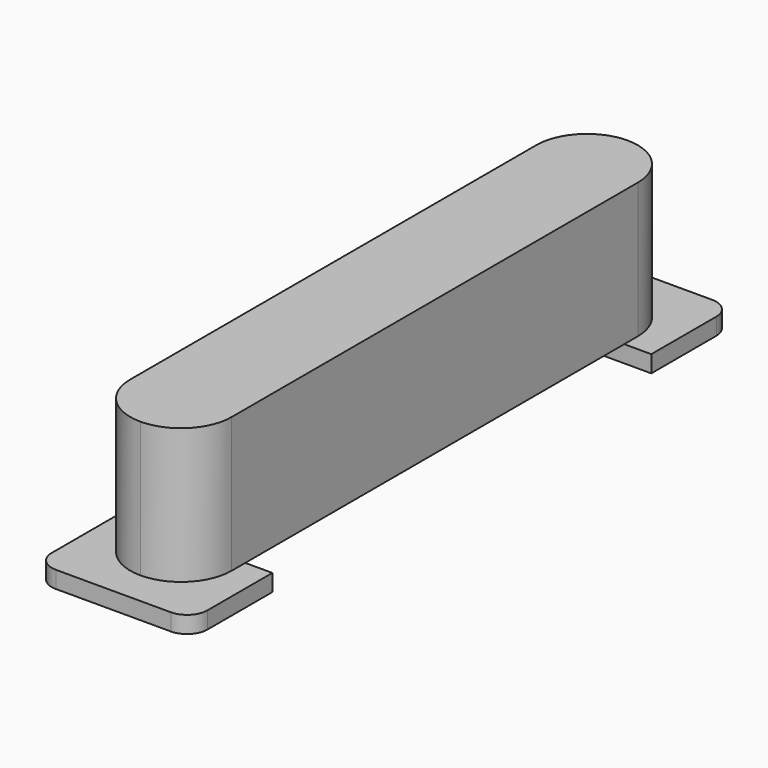
from build123d import *

# Parameters (mm, degrees)
F0_W     = 1.5
F0_H     = 1
F0_H_2   = 7
F1_DEPTH = 2
F2_DEPTH = 0.25
F3_R     = 0.74999
F4_R     = 0.3


# Not quite as in the source:
# - a fillet or chamfer is up to 0.001 mm smaller than in the source, because OpenCascade refuses the exact size
# - a feature names something its author has since deleted; it is built from what else it names


with BuildPart() as f1:
    # F0 (on Top) → F1 (new body)
    with BuildSketch(Plane.XY):
        with Locations((-0.75, 9.1787409857)):
            Rectangle(F0_W, F0_H)
        with Locations((-0.75, 5.1787409857)):
            Rectangle(F0_W, F0_H_2)
        with Locations((-0.75, 1.1787409857)):
            Rectangle(F0_W, F0_H)
    extrude(amount=F1_DEPTH)

    # F0 (on Top) → F2 (join)
    with BuildSketch(Plane.XY):
        with Locations((-0.75, 1.1787409857)):
            Rectangle(F0_W, F0_H)
        Polygon((-1.5, 0.6787409857), (-1.5, 1.6787409857), (-1.9, 1.6787409857), (-1.9, 0.1787409857), (0.4, 0.1787409857), (0.4, 1.6787409857), (0, 1.6787409857), (0, 0.6787409857), align=None)
        Polygon((-1.5, 8.6787409857), (-1.5, 9.6787409857), (0, 9.6787409857), (0, 8.6787409857), (0.4, 8.6787409857), (0.4, 10.1787409857), (-1.9, 10.1787409857), (-1.9, 8.6787409857), align=None)
        with Locations((-0.75, 9.1787409857)):
            Rectangle(F0_W, F0_H)
    extrude(amount=-F2_DEPTH)

    # F3 (radius 0.75 in the source; OpenCascade refuses exactly that, so slightly less here)
    f3_edges = [f1.edges().sort_by_distance(p)[0] for p in [
        (0, 9.678741, 1),
        (-1.5, 9.678741, 1),
        (0, 0.678741, 1),
        (-1.5, 0.678741, 1),
    ]]
    fillet(f3_edges, radius=F3_R)

    # F4
    f4_edges = [f1.edges().sort_by_distance(p)[0] for p in [
        (0.4, 10.178741, -0.125),
        (-1.9, 10.178741, -0.125),
        (0.4, 0.178741, -0.125),
        (-1.9, 0.178741, -0.125),
    ]]
    fillet(f4_edges, radius=F4_R)


solid = f1.part
